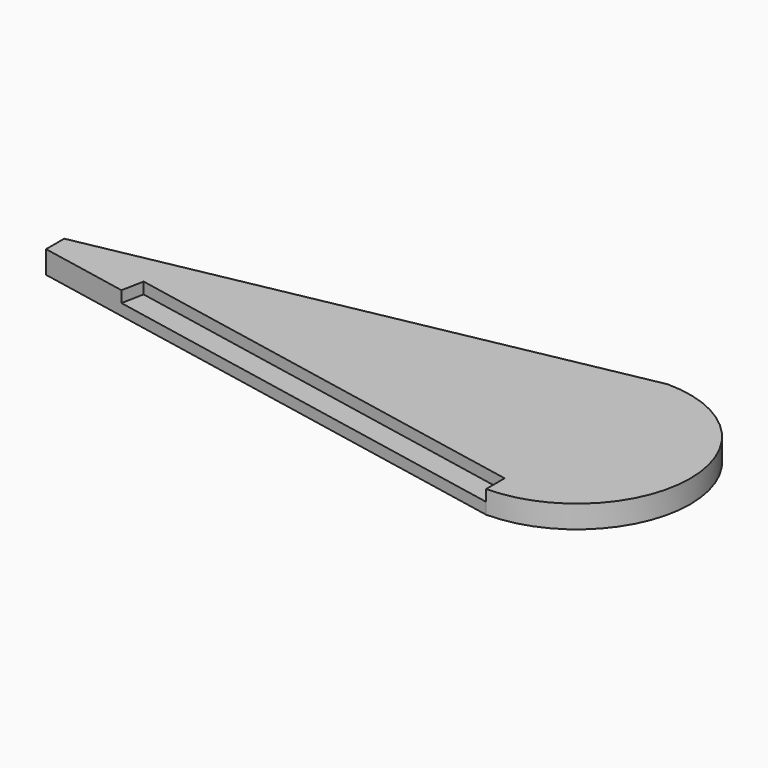
from build123d import *

# Parameters (mm, degrees)
F0_W     = 177.8
F0_H     = 63.5
F1_DEPTH = 6.35
F3_DEPTH = 25.4
F5_DEPTH = 25.4
F6_R     = 3.1115
F7_DEPTH = 25.4
F9_DEPTH = 3.175


# Not quite as in the source:
# - ends of sketch curves that miss each other by under 0.0002 mm in the source are joined


with BuildPart() as f1:
    # F0 (on Top) → F1 (new body)
    with BuildSketch(Plane.XY):
        with Locations((88.9, 31.75)):
            Rectangle(F0_W, F0_H)
    extrude(amount=F1_DEPTH)

    # F2 (on face) → F3 (cut)
    with BuildSketch(Plane.XY.offset(6.35)):
        with BuildLine():
            ThreePointArc((146.05, 63.5), (168.5006403027, 54.2006403027), (177.8, 31.75))
            Line((177.8, 31.75), (177.8, 63.5))
            Line((177.8, 63.5), (146.05, 63.5))
        make_face()
        with BuildLine():
            ThreePointArc((177.8, 31.75), (168.5006402649, 9.2993596596), (146.0499998933, 0))
            Line((146.0499998933, 0), (177.8, 0))
            Line((177.8, 0), (177.8, 31.75))
        make_face()
    extrude(amount=-F3_DEPTH, mode=Mode.SUBTRACT)

    # F4 (on face) → F5 (cut)
    with BuildSketch(Plane.XY.offset(6.35)):
        Polygon((0, 34.925), (146.05, 63.5), (0, 63.5), align=None)
        Polygon((0, 0), (146.0499998933, 0), (0, 28.575), align=None)
    extrude(amount=-F5_DEPTH, mode=Mode.SUBTRACT)

    # F6 (on face) → F7 (cut)
    with BuildSketch(Plane(origin=(0, 0, 0), x_dir=(0, -1, 0), z_dir=(-1, 0, 0))):
        with Locations((-31.75, 3.175)):
            Circle(F6_R)
    extrude(amount=-F7_DEPTH, mode=Mode.SUBTRACT)

    # F8 (on face) → F9 (cut)
    with BuildSketch(Plane.XY.offset(6.35)):
        Polygon((26.2400177438, 29.9114803934), (25.0207440433, 23.679637035), (146.05, 0), (146.05, 6.4703969085), align=None)
    extrude(amount=-F9_DEPTH, mode=Mode.SUBTRACT)


solid = f1.part
